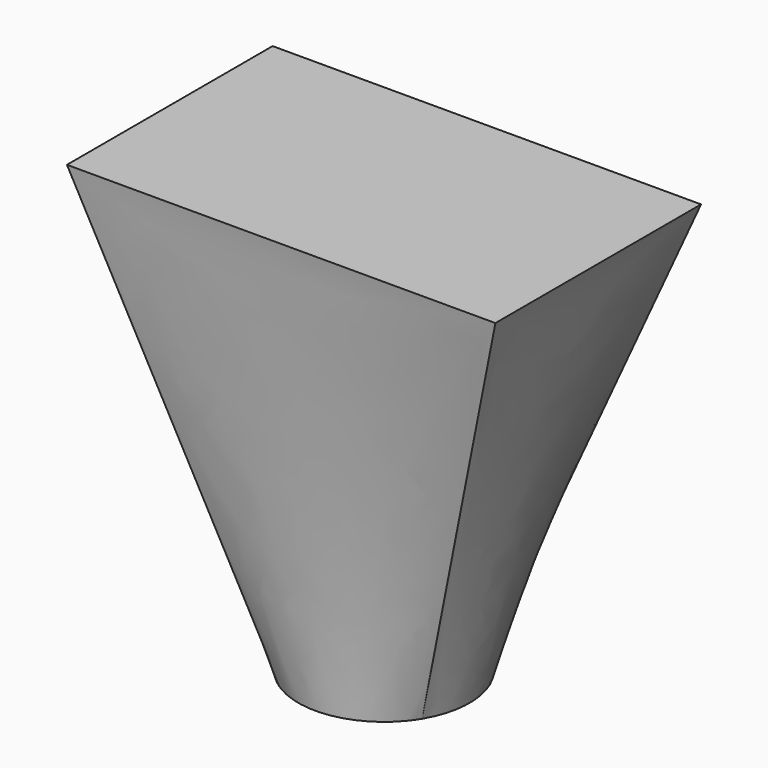
from build123d import *

# Parameters (mm, degrees)
F2_W = 127
F2_H = 76.2


# Not quite as in the source:
# - the arcs of a loft's sections are written as splines that run evenly, so that the points pair up as in the source's solid


with BuildPart() as f3:
    # F2 (on offset) → F3 section 0
    with BuildSketch(Plane.XY.offset(127)):
        Rectangle(F2_W, F2_H)
    # F1 (on Top) → F3 section 1
    with BuildSketch(Plane.XY):
        with BuildLine():
            add(Edge.make_bspline(
                [(-21.7803203131, 13.0681921879), (-22.6356314917, 11.6426735568), (-23.3505236623, 10.1329514593), (-24.472067113, 7.0029702123), (-24.8786906608, 5.3827884578), (-25.3680549193, 2.0941466499), (-25.4507835294, 0.4257679146), (-25.2891626016, -2.8951537939), (-25.04481706, -4.5476146508), (-24.2384219474, -7.773195101), (-23.6763923162, -9.3462349355), (-22.2562123309, -12.3525168797), (-21.3980970935, -13.7856846531), (-19.4187089559, -16.457138362), (-18.2974849998, -17.6953582406), (-15.8349554859, -19.9293212464), (-14.4937108189, -20.9250091345), (-13.0681921879, -21.7803203131)],
                knots=[0, 0, 0, 0, 0.125, 0.125, 0.25, 0.25, 0.375, 0.375, 0.5, 0.5, 0.625, 0.625, 0.75, 0.75, 0.875, 0.875, 1, 1, 1, 1], degree=3))
            add(Edge.make_bspline(
                [(-13.0681921879, -21.7803203131), (-11.6426735568, -22.6356314917), (-10.1329514593, -23.3505236623), (-7.0029702123, -24.472067113), (-5.3827884578, -24.8786906608), (-2.0941466499, -25.3680549193), (-0.4257679146, -25.4507835294), (2.8951537939, -25.2891626016), (4.5476146508, -25.04481706), (7.773195101, -24.2384219474), (9.3462349355, -23.6763923162), (12.3525168797, -22.2562123309), (13.7856846531, -21.3980970935), (16.457138362, -19.4187089559), (17.6953582406, -18.2974849998), (19.9293212464, -15.8349554859), (20.9250091345, -14.4937108189), (21.7803203131, -13.0681921879)],
                knots=[0, 0, 0, 0, 0.125, 0.125, 0.25, 0.25, 0.375, 0.375, 0.5, 0.5, 0.625, 0.625, 0.75, 0.75, 0.875, 0.875, 1, 1, 1, 1], degree=3))
            add(Edge.make_bspline(
                [(21.7803203131, -13.0681921879), (22.6356314917, -11.6426735568), (23.3505236623, -10.1329514593), (24.472067113, -7.0029702123), (24.8786906608, -5.3827884578), (25.3680549193, -2.0941466499), (25.4507835294, -0.4257679146), (25.2891626016, 2.8951537939), (25.04481706, 4.5476146508), (24.2384219474, 7.773195101), (23.6763923162, 9.3462349355), (22.2562123309, 12.3525168797), (21.3980970935, 13.7856846531), (19.4187089559, 16.457138362), (18.2974849998, 17.6953582406), (15.8349554859, 19.9293212464), (14.4937108189, 20.9250091345), (13.0681921879, 21.7803203131)],
                knots=[0, 0, 0, 0, 0.125, 0.125, 0.25, 0.25, 0.375, 0.375, 0.5, 0.5, 0.625, 0.625, 0.75, 0.75, 0.875, 0.875, 1, 1, 1, 1], degree=3))
            add(Edge.make_bspline(
                [(13.0681921879, 21.7803203131), (11.6426735568, 22.6356314917), (10.1329514593, 23.3505236623), (7.0029702123, 24.472067113), (5.3827884578, 24.8786906608), (2.0941466499, 25.3680549193), (0.4257679146, 25.4507835294), (-2.8951537939, 25.2891626016), (-4.5476146508, 25.04481706), (-7.773195101, 24.2384219474), (-9.3462349355, 23.6763923162), (-12.3525168797, 22.2562123309), (-13.7856846531, 21.3980970935), (-16.457138362, 19.4187089559), (-17.6953582406, 18.2974849998), (-19.9293212464, 15.8349554859), (-20.9250091345, 14.4937108189), (-21.7803203131, 13.0681921879)],
                knots=[0, 0, 0, 0, 0.125, 0.125, 0.25, 0.25, 0.375, 0.375, 0.5, 0.5, 0.625, 0.625, 0.75, 0.75, 0.875, 0.875, 1, 1, 1, 1], degree=3))
        make_face()
    loft(ruled=True)


solid = f3.part
